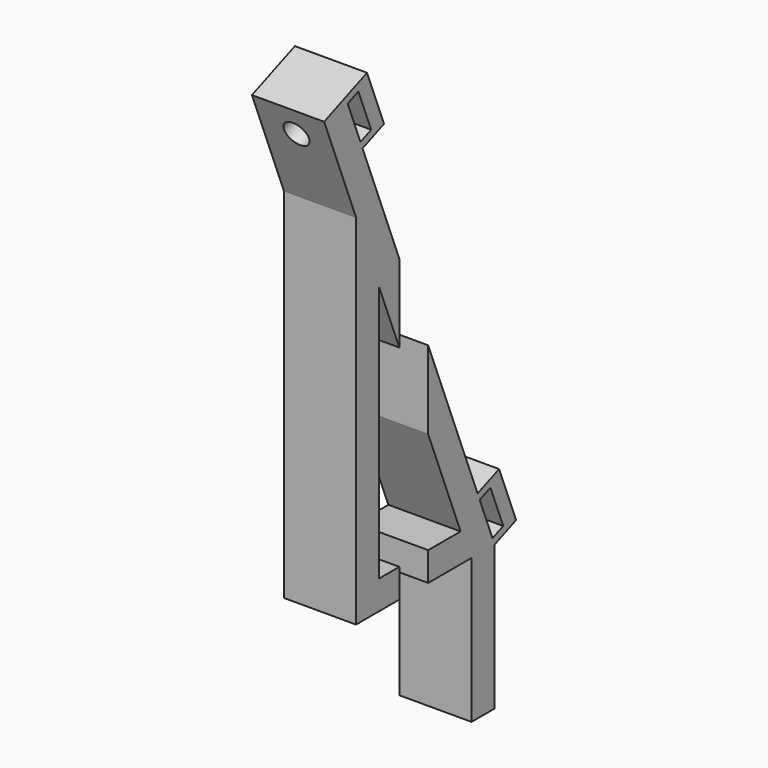
from build123d import *

# Parameters (mm, degrees)
F1_DEPTH = 10
F2_R     = 1.75
F3_DEPTH = 25
F4_R     = 1.75
F5_DEPTH = 6.5
F6_W     = 7.5
F6_H     = 5
F7_DEPTH = 52.6


with BuildPart() as f1:
    # F0 (on Right) → F1 (new body)
    with BuildSketch(Plane.YZ):
        Polygon((-20, 49.6487663492), (-20, 0), (0, 0), (0, -20), (4, -20), (4, 0), (3.6312381011, 0.9295238899), (1.4186667076, 6.5066672293), (1.0499048087, 7.4361911193), (-18.8632377328, 57.6304811742), (-19.2319996317, 58.5600050641), (-21.4445710252, 64.1371484036), (-21.8133329241, 65.0666722935), (-25.5314284837, 63.5916246978), align=None)
        Polygon((-16, 4), (-16, 39.5661206894), (-1.8901633999, 4), align=None, mode=Mode.SUBTRACT)
        Polygon((-18.0952373645, 66.5417198892), (-21.8133329241, 65.0666722935), (-21.4445710252, 64.1371484036), (-19.5855232454, 64.8746722014), (-17.3729518519, 59.297528862), (-19.2319996317, 58.5600050641), (-18.8632377328, 57.6304811742), (-15.1451421732, 59.1055287699), align=None)
        Polygon((3.6312381011, 0.9295238899), (4, 0), (7.7180955596, 1.4750475957), (4.7680003683, 8.9112387149), (1.0499048087, 7.4361911193), (1.4186667076, 6.5066672293), (3.2777144874, 7.2441910272), (5.4902858809, 1.6670476877), align=None)
    extrude(amount=F1_DEPTH)

    # F2 (on face) → F3 (cut)
    with BuildSketch(Plane(origin=(0, 7.1741542073, 2.8461395746), x_dir=(-1, 0, 0), z_dir=(0, 0.9295238899, 0.3687618989))):
        with Locations((-5, 64.5249524043)):
            Circle(F2_R)
    extrude(amount=-F3_DEPTH, mode=Mode.SUBTRACT)

    # F4 (on face) → F5 (cut)
    with BuildSketch(Plane(origin=(0, 7.1741542073, 2.8461395746), x_dir=(-1, 0, 0), z_dir=(0, 0.9295238899, 0.3687618989))):
        with Locations((-5, 2.5249524043)):
            Circle(F4_R)
    extrude(amount=-F5_DEPTH, mode=Mode.SUBTRACT)

    # F6 (on face) → F7 (cut)
    with BuildSketch(Plane(origin=(0, 0, 0), x_dir=(1, 0, 0), z_dir=(0, 0, -1))):
        with Locations((6.25, 10)):
            Rectangle(F6_W, F6_H)
    extrude(amount=-F7_DEPTH, mode=Mode.SUBTRACT)


solid = f1.part
